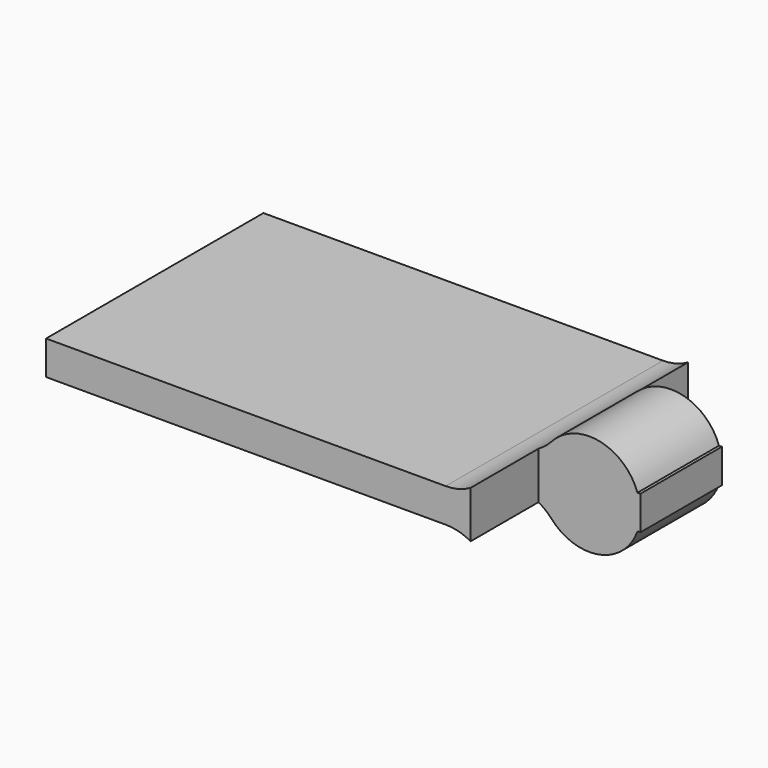
from build123d import *

# Parameters (mm, degrees)
F0_W     = 3
F0_H     = 6
F3_DEPTH = 1
F4_D     = 1
F6_R     = 3


with BuildPart() as f2:
    # F0 (on Top) → F2 (revolve)
    with BuildSketch(Plane.XY):
        with Locations((1.5, 8)):
            Rectangle(F0_W, F0_H)
    revolve(axis=Axis((0, 8, 0), (0, -1, 0)))

    # F4 (through all)
    with Locations(Plane.XZ):
        with Locations((0, 0)):
            Hole(F4_D / 2)


with BuildPart() as f3:
    # F0 (on Top) → F3 (new body, symmetric)
    with BuildSketch(Plane.XY):
        Polygon((-28, 16), (-28, 0), (-3, 0), (-3, 5), (0, 5), (0, 11), (-3, 11), (-3, 16), align=None)
        with Locations((1.5, 8)):
            Rectangle(F0_W, F0_H)
    extrude(amount=F3_DEPTH, both=True)


with BuildPart() as f2_1:
    add(f2.part)

    # F5: union F3
    add(f3.part)

    # F6 (call 1 of 2: OpenCascade refuses the feature's edges together)
    f6_edges = [f2_1.edges().sort_by_distance(p)[0] for p in [
        (-2.828427, 8, 1),
    ]]
    fillet(f6_edges, radius=F6_R)

    # F6#2 (call 2 of 2)
    f6_2_edges = [f2_1.edges().sort_by_distance(p)[0] for p in [
        (-2.828427, 8, -1),
    ]]
    fillet(f6_2_edges, radius=F6_R)


solid = f2_1.part
